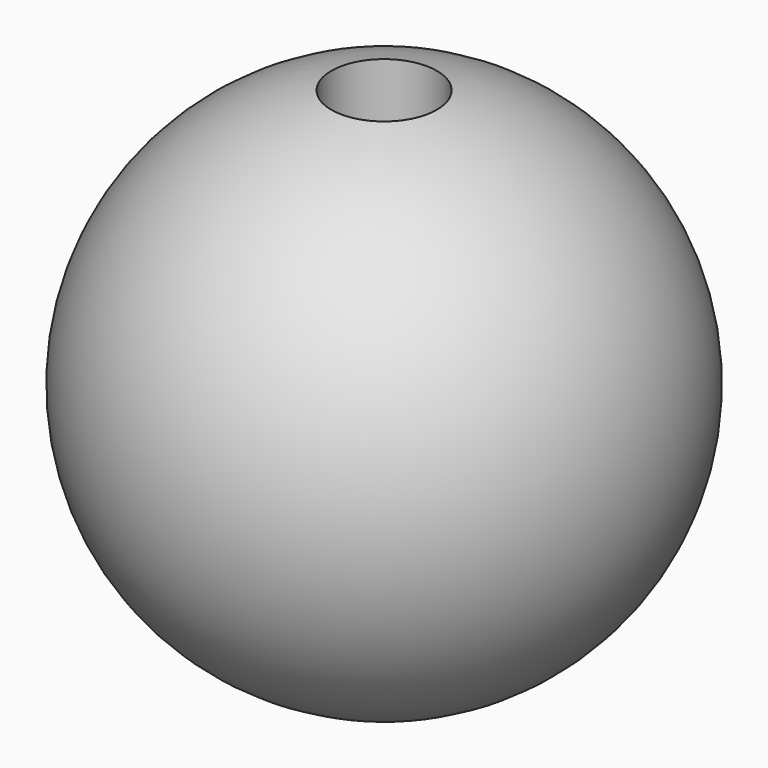
from build123d import *

# Parameters (mm, degrees)
F4_R     = 3.175
F5_DEPTH = 50.8


# Not quite as in the source:
# - a length typed as a fraction of an inch, garbled in the dataset ("3 / 203.2 mm" for 3/8 in), is restored


with BuildPart() as f2:
    # F0 (on Front) → F2 (revolve)
    with BuildSketch(Plane.XZ):
        with BuildLine():
            Line((0, -15.875), (0, 15.875))
            ThreePointArc((0, 15.875), (-15.875, 0), (0, -15.875))
        make_face()
    revolve(axis=Axis((0, 0, 0), (0, 0, 1)))


with BuildPart() as f5:
    # F4 (on offset) → F5 (new body)
    with BuildSketch(Plane.XY.offset(6.35)):
        Circle(F4_R)
    extrude(amount=F5_DEPTH)


with BuildPart() as f2_1:
    add(f2.part)

    # F6: cut F5
    add(f5.part, mode=Mode.SUBTRACT)


solid = f2_1.part
